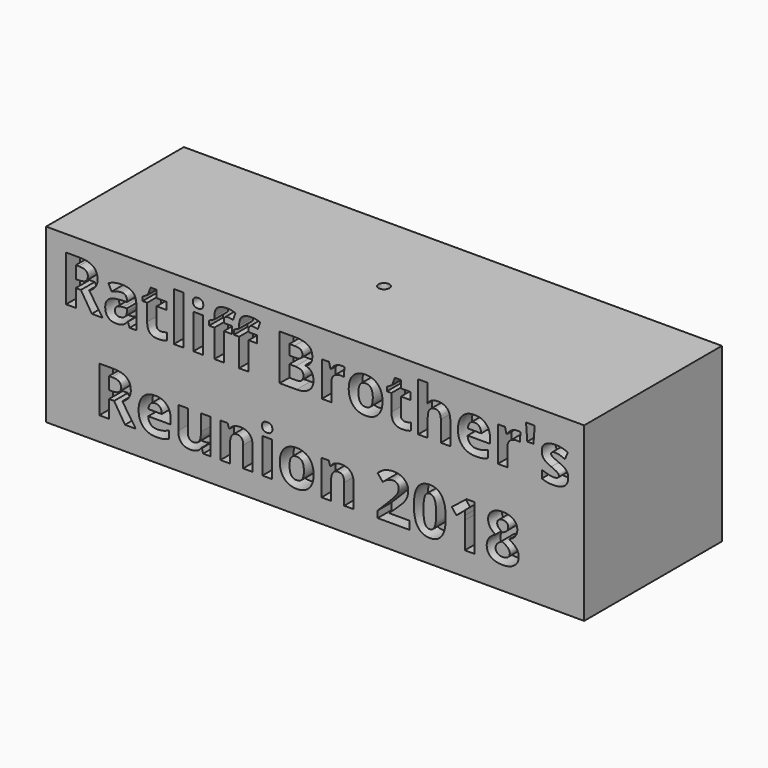
from build123d import *

# Parameters (mm, degrees)
F0_W         = 79.375
F0_H         = 25.4
F1_DEPTH     = 12.7
F2_TEXT_SIZE = 9.424028556
F3_DEPTH     = 2.54
F4_R         = 0.79375
F5_DEPTH     = 12.7


# Not quite as in the source:
# - Text() gives the source's letters only with a copy of the font that has no kerning and outlines rounded to 1/6400 em; it was checked with that copy


with BuildPart() as f1:
    # F0 (on Top) → F1 (new body, symmetric)
    with BuildSketch(Plane.XY):
        Rectangle(F0_W, F0_H)
    extrude(amount=F1_DEPTH, both=True)

    # F2 (on face) → F3 (cut)
    with BuildSketch(Plane.XZ.offset(12.7)):
        with Locations((-37.5819733739, 3.5630627535)):
            Text("Ratliff Brother's", F2_TEXT_SIZE, font='Open Sans', font_style=FontStyle.BOLD, text_align=(TextAlign.LEFT, TextAlign.BOTTOM))
        with Locations((-32.6844235337, -9.2536160826)):
            Text('Reunion 2018', F2_TEXT_SIZE, font='Open Sans', font_style=FontStyle.BOLD, text_align=(TextAlign.LEFT, TextAlign.BOTTOM))
    extrude(amount=-F3_DEPTH, mode=Mode.SUBTRACT)

    # F4 (on face) → F5 (cut)
    with BuildSketch(Plane.XY.offset(12.7)):
        Circle(F4_R)
    extrude(amount=-F5_DEPTH, mode=Mode.SUBTRACT)


solid = f1.part
